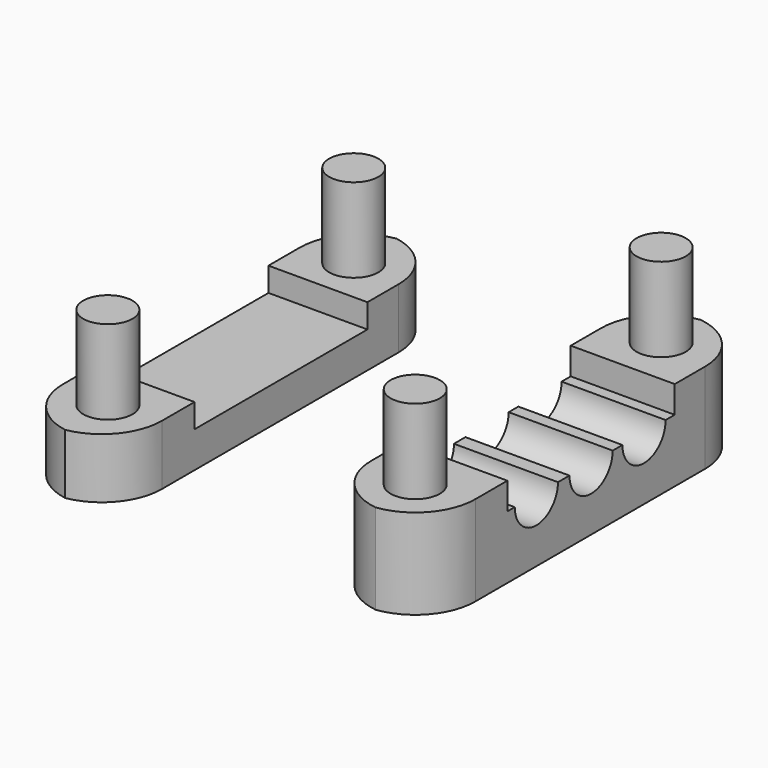
from build123d import *

# Parameters (mm, degrees)
F0_W         = 8.2438504323
F0_H         = 34.6492690086
F1_DEPTH     = 5
F2_R         = 2.05
F3_DEPTH     = 12
F5_DEPTH     = 12.5
F6_T1_DEPTH  = 30
F7_W         = 8.6631612957
F7_H         = 33.9300383866
F7_R         = 2.05
F8_DEPTH     = 7.5
F9_DEPTH     = 14.5
F10_T1_DEPTH = 32.5
F12_DEPTH    = 29.9325806478


# Not quite as in the source:
# - a fillet or chamfer that OpenCascade refuses, or shapes differently, is made with other operations: its cross-section is extruded or revolved along the edge and cut away or added


with BuildPart() as f1:
    # F0 (on Top) → F1 (new body)
    with BuildSketch(Plane.XY):
        with Locations((0, -12.8)):
            Rectangle(F0_W, F0_H)
        with BuildLine():
            ThreePointArc((1.9, -25.6), (-1.3435028843, -26.9435028843), (0, -23.7))
            ThreePointArc((0, -23.7), (1.3435028843, -24.2564971157), (1.9, -25.6))
        make_face(mode=Mode.SUBTRACT)
        with BuildLine():
            ThreePointArc((0, -1.9), (-1.3435028843, 1.3435028843), (1.9, 0))
            ThreePointArc((1.9, 0), (1.3435028843, -1.3435028843), (0, -1.9))
        make_face(mode=Mode.SUBTRACT)
        with BuildLine():
            ThreePointArc((0, -1.9), (1.3435028843, -1.3435028843), (1.9, 0))
            ThreePointArc((1.9, 0), (-1.3435028843, 1.3435028843), (0, -1.9))
        make_face()
        with BuildLine():
            ThreePointArc((1.9, -25.6), (1.3435028843, -24.2564971157), (0, -23.7))
            ThreePointArc((0, -23.7), (-1.3435028843, -26.9435028843), (1.9, -25.6))
        make_face()
    extrude(amount=F1_DEPTH)

    # F2 (on Top) → F3 (join)
    with BuildSketch(Plane.XY):
        Circle(F2_R)
        with Locations((0, -25.5993018519)):
            Circle(F2_R)
    extrude(amount=F3_DEPTH)

    # F4 (on Right) → F5 (cut, symmetric)
    with BuildSketch(Plane.YZ):
        Polygon((-21.728410773, 3), (-12.728410773, 3), (-3.728410773, 3), (-3.728410773, 5), (-21.728410773, 5), align=None)
    extrude(amount=F5_DEPTH, both=True, mode=Mode.SUBTRACT)

    # F6: fillet of radius 5 on 4 edges, made by hand

    # F6_s2 → F6_t1 (cut)
    with BuildSketch(Plane.XY.offset(-12.5)):
        with BuildLine():
            ThreePointArc((-0.8780747838, 4.5246345043), (2.6574591221, 3.0601684103), (4.1219252162, -0.4753654957))
            Line((4.1219252162, -0.4753654957), (4.1219252162, 4.5246345043))
            Line((4.1219252162, 4.5246345043), (-0.8780747838, 4.5246345043))
        make_face()
        with BuildLine():
            ThreePointArc((-4.1219252162, -0.4753654957), (-2.6574591221, 3.0601684103), (0.8780747838, 4.5246345043))
            Line((0.8780747838, 4.5246345043), (-4.1219252162, 4.5246345043))
            Line((-4.1219252162, 4.5246345043), (-4.1219252162, -0.4753654957))
        make_face()
        with BuildLine():
            ThreePointArc((-4.1219252162, -25.1246345043), (-2.6574591221, -28.6601684103), (0.8780747838, -30.1246345043))
            Line((0.8780747838, -30.1246345043), (-4.1219252162, -30.1246345043))
            Line((-4.1219252162, -30.1246345043), (-4.1219252162, -25.1246345043))
        make_face()
        with BuildLine():
            ThreePointArc((-0.8780747838, -30.1246345043), (2.6574591221, -28.6601684103), (4.1219252162, -25.1246345043))
            Line((4.1219252162, -25.1246345043), (4.1219252162, -30.1246345043))
            Line((4.1219252162, -30.1246345043), (-0.8780747838, -30.1246345043))
        make_face()
    extrude(amount=F6_T1_DEPTH, mode=Mode.SUBTRACT)


with BuildPart() as f8:
    # F7 (on Top) → F8 (new body)
    with BuildSketch(Plane.XY):
        with Locations((25.6, -12.8)):
            Rectangle(F7_W, F7_H)
        with Locations((25.6, -25.6)):
            Circle(F7_R, mode=Mode.SUBTRACT)
        with Locations((25.6, 0)):
            Circle(F7_R, mode=Mode.SUBTRACT)
        with Locations((25.6, -25.6)):
            Circle(F7_R)
        with Locations((25.6, 0)):
            Circle(F7_R)
    extrude(amount=F8_DEPTH)

    # F7 (on Top) → F9 (join)
    with BuildSketch(Plane.XY):
        with Locations((25.6, 0)):
            Circle(F7_R)
        with Locations((25.6, -25.6)):
            Circle(F7_R)
    extrude(amount=F9_DEPTH)

    # F10: fillet of radius 5 on 4 edges, made by hand

    # F10_s2 → F10_t1 (cut)
    with BuildSketch(Plane.XY.offset(-12.5)):
        with BuildLine():
            ThreePointArc((24.9315806478, 4.1650191933), (28.4671145538, 2.7005530992), (29.9315806478, -0.8349808067))
            Line((29.9315806478, -0.8349808067), (29.9315806478, 4.1650191933))
            Line((29.9315806478, 4.1650191933), (24.9315806478, 4.1650191933))
        make_face()
        with BuildLine():
            ThreePointArc((24.9315806478, -29.7650191933), (28.4671145538, -28.3005530992), (29.9315806478, -24.7650191933))
            Line((29.9315806478, -24.7650191933), (29.9315806478, -29.7650191933))
            Line((29.9315806478, -29.7650191933), (24.9315806478, -29.7650191933))
        make_face()
        with BuildLine():
            ThreePointArc((21.2684193522, -24.7650191933), (22.7328854462, -28.3005530992), (26.2684193522, -29.7650191933))
            Line((26.2684193522, -29.7650191933), (21.2684193522, -29.7650191933))
            Line((21.2684193522, -29.7650191933), (21.2684193522, -24.7650191933))
        make_face()
        with BuildLine():
            ThreePointArc((21.2684193522, -0.8349808067), (22.7328854462, 2.7005530992), (26.2684193522, 4.1650191933))
            Line((26.2684193522, 4.1650191933), (21.2684193522, 4.1650191933))
            Line((21.2684193522, 4.1650191933), (21.2684193522, -0.8349808067))
        make_face()
    extrude(amount=F10_T1_DEPTH, mode=Mode.SUBTRACT)

    # F11 (on Right) → F12 (cut, through all)
    with BuildSketch(Plane.YZ):
        with BuildLine():
            Line((-4.9487714618, 5.25), (-4, 5.25))
            Line((-4, 5.25), (-4, 7.5))
            Line((-4, 7.5), (-21.4204657823, 7.5))
            Line((-21.4204657823, 7.5), (-21.4204657823, 5.25))
            Line((-21.4204657823, 5.25), (-20.6557280421, 5.25))
            ThreePointArc((-20.6557280421, 5.25), (-18.4057280421, 3), (-16.1557280421, 5.25))
            Line((-16.1557280421, 5.25), (-14.9602328911, 5.25))
            ThreePointArc((-14.9602328911, 5.25), (-12.7102328911, 3), (-10.4602328911, 5.25))
            Line((-10.4602328911, 5.25), (-9.4487714618, 5.25))
            ThreePointArc((-9.4487714618, 5.25), (-7.1987714618, 3), (-4.9487714618, 5.25))
        make_face()
    extrude(amount=F12_DEPTH, mode=Mode.SUBTRACT)


solid = Compound([f1.part, f8.part])
